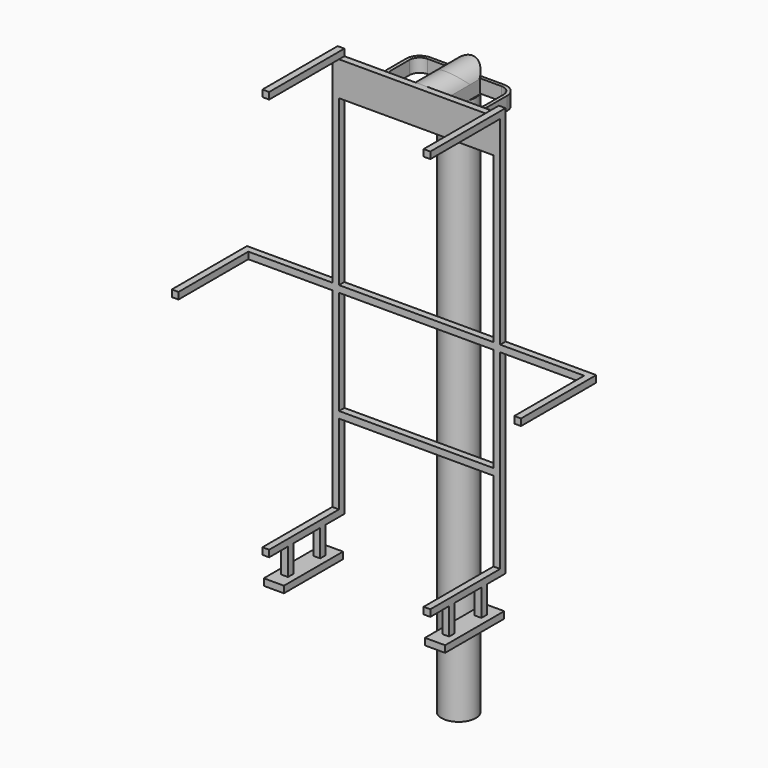
from build123d import *
from build123d import SkipClean  # not in build123d's __all__

# Parameters (mm, degrees)
F0_R      = 25.5
F1_DEPTH  = 850
F2_R      = 25.5
F3_DEPTH  = 69
F5_DEPTH  = 150
F7_DEPTH  = 75
F8_R      = 20
F10_DEPTH = 20
F12_DEPTH = 10
F13_W     = 230
F13_H     = 155
F14_DEPTH = 10
F16_W     = 10
F16_H     = 130
F16_H_2   = 10
F17_DEPTH = 10
F15_W     = 10
F15_H     = 10
F18_DEPTH = 130
F19_W     = 10
F19_H     = 10
F20_DEPTH = 40
F21_W     = 10
F21_H     = 10
F22_DEPTH = 10


with BuildPart() as f1:
    # F0 (on Top) → F1 (new body)
    with BuildSketch(Plane.XY):
        Circle(F0_R)
    extrude(amount=F1_DEPTH)

    # F2 (on Front) → F3 (join)
    with BuildSketch(Plane.XZ):
        with Locations((0, 824.5)):
            Circle(F2_R)
    with SkipClean():  # cleaning this boolean's faces spoils the solid; the shape is the same uncleaned
        extrude(amount=F3_DEPTH)

    # F4 (on face) → F5 (cut)
    with BuildSketch(Plane.XZ.offset(69)):
        with BuildLine():
            ThreePointArc((-25.5, 824.5), (0, 850), (25.5, 824.5))
            Line((25.5, 824.5), (45.5921813846, 824.5))
            Line((45.5921813846, 824.5), (45.5921813846, 859.704375267))
            Line((45.5921813846, 859.704375267), (-40.7917350531, 859.704375267))
            Line((-40.7917350531, 859.704375267), (-40.7917350531, 824.5))
            Line((-40.7917350531, 824.5), (-25.5, 824.5))
        make_face()
    extrude(amount=-F5_DEPTH, mode=Mode.SUBTRACT)

    # F6 (on Right) → F7 (join, symmetric)
    with BuildSketch(Plane.YZ):
        Polygon((-59, 833.4226703644), (-59, 823.4226703644), (-59, 813.4226703644), (16, 813.4226703644), (16, 833.4226703644), align=None)
    extrude(amount=F7_DEPTH, both=True)

    # F8
    f8_edges = [f1.edges().sort_by_distance(p)[0] for p in [
        (75, 16, 823.42267),
        (-75, 16, 823.42267),
        (-75, -59, 823.42267),
        (75, -59, 823.42267),
    ]]
    fillet(f8_edges, radius=F8_R)

    # F9 (on face) → F10 (cut)
    with BuildSketch(Plane.XY.offset(833.4226703644)):
        with BuildLine():
            Line((-23.8879876417, -54), (-23.8879876417, 8.9226703644))
            Line((-23.8879876417, 8.9226703644), (-23.0054341407, 11))
            Line((-23.0054341407, 11), (-55, 11))
            ThreePointArc((-55, 11), (-65.6066017178, 6.6066017178), (-70, -4))
            Line((-70, -4), (-70, -39))
            ThreePointArc((-70, -39), (-65.6066017178, -49.6066017178), (-55, -54))
            Line((-55, -54), (-23.8879876417, -54))
        make_face()
        with BuildLine():
            Line((23.8879876417, -8.9226703644), (23.8879876417, -54))
            Line((23.8879876417, -54), (55, -54))
            ThreePointArc((55, -54), (65.6066017178, -49.6066017178), (70, -39))
            Line((70, -39), (70, -4))
            ThreePointArc((70, -4), (65.6066017178, 6.6066017178), (55, 11))
            Line((55, 11), (23.0054341407, 11))
            ThreePointArc((23.0054341407, 11), (23.4697054992, 9.9711044415), (23.8879876417, 8.9226703644))
            Line((23.8879876417, 8.9226703644), (23.8879876417, -8.9226703644))
        make_face()
    extrude(amount=-F10_DEPTH, mode=Mode.SUBTRACT)


with BuildPart() as f12:
    # F11 (on face) → F12 (new body)
    with BuildSketch(Plane.XZ.offset(69)):
        Polygon((125, 554), (125, 850), (-125, 850), (-125, 554), (-260, 554), (-260, 544), (-125, 544), (-125, 250), (-115, 250), (-115, 379), (0, 379), (115, 379), (115, 250), (125, 250), (125, 544), (260, 544), (260, 554), align=None)
    extrude(amount=F12_DEPTH)

    # F13 (on face) → F14 (cut)
    with BuildSketch(Plane.XZ.offset(79)):
        Polygon((115, 799), (0, 799), (-115, 799), (-115, 554), (115, 554), align=None)
        with Locations((0, 466.5)):
            Rectangle(F13_W, F13_H)
    extrude(amount=-F14_DEPTH, mode=Mode.SUBTRACT)

    # F16 (on face) → F17 (join)
    with BuildSketch(Plane.XY.offset(850)):
        with Locations((-120, -144)):
            Rectangle(F16_W, F16_H)
        with Locations((120, -74)):
            Rectangle(F16_W, F16_H_2)
        with Locations((-120, -74)):
            Rectangle(F16_W, F16_H_2)
        with Locations((120, -144)):
            Rectangle(F16_W, F16_H)
    extrude(amount=F17_DEPTH)

    # F15 (on face) → F18 (join)
    with BuildSketch(Plane.XZ.offset(79)):
        with Locations((-255, 549)):
            Rectangle(F15_W, F15_H)
        with Locations((255, 549)):
            Rectangle(F15_W, F15_H)
        with Locations((120, 255)):
            Rectangle(F15_W, F15_H)
        with Locations((-120, 255)):
            Rectangle(F15_W, F15_H)
    extrude(amount=F18_DEPTH)

    # F19 (on face) → F20 (join)
    with BuildSketch(Plane(origin=(0, 0, 250), x_dir=(1, 0, 0), z_dir=(0, 0, -1))):
        with Locations((-120, 109)):
            Rectangle(F19_W, F19_H)
        with Locations((-120, 169)):
            Rectangle(F19_W, F19_H)
        with Locations((120, 169)):
            Rectangle(F19_W, F19_H)
        with Locations((120, 109)):
            Rectangle(F19_W, F19_H)
    extrude(amount=F20_DEPTH)

    # F21 (on face) → F22 (join)
    with BuildSketch(Plane(origin=(0, 0, 210), x_dir=(1, 0, 0), z_dir=(0, 0, -1))):
        Polygon((-135, 194), (-135, 104), (-135, 84), (-105, 84), (-105, 194), align=None)
        with Locations((-120, 109)):
            Rectangle(F21_W, F21_H, mode=Mode.SUBTRACT)
        Polygon((105, 84), (135, 84), (135, 104), (135, 194), (105, 194), align=None)
        with Locations((-120, 109)):
            Rectangle(F21_W, F21_H)
    extrude(amount=F22_DEPTH)


solid = Compound([f1.part, f12.part])
